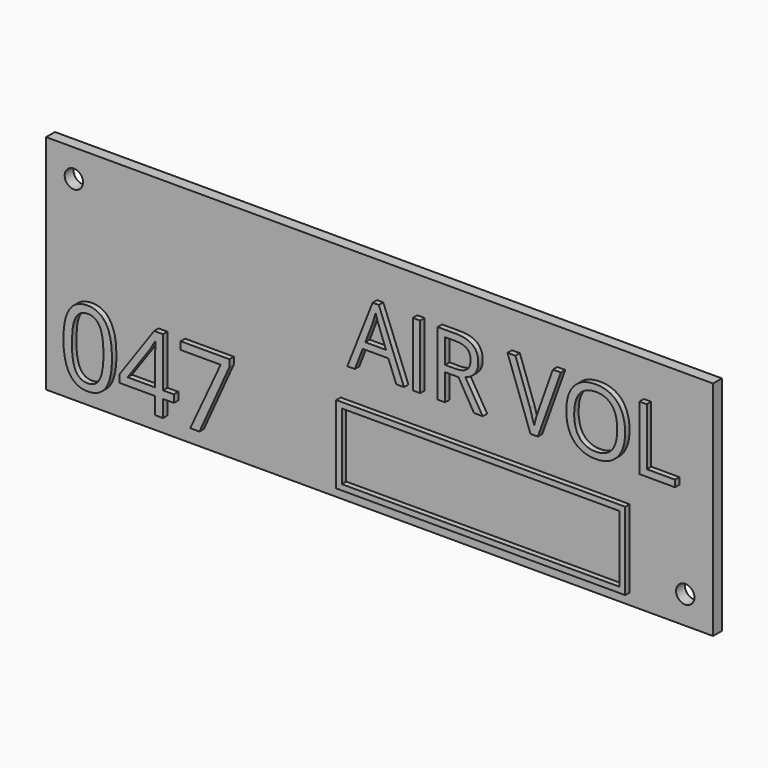
from build123d import *

# Parameters (mm, degrees)
F0_W         = 120
F0_H         = 40
F1_DEPTH     = 2
F3_D         = 3.3
F4_TEXT_SIZE = 16.1100855848
F5_DEPTH     = 1
F6_TEXT_SIZE = 18.5054667028
F7_DEPTH     = 1
F8_W         = 52
F8_H         = 14
F8_W_2       = 49.99999962
F8_H_2       = 11.99999962
F9_DEPTH     = 1


# Not quite as in the source:
# - Text() gives the source's letters only with a copy of the font that has no kerning and outlines rounded to 1/6400 em; it was checked with that copy


with BuildPart() as f1:
    # F0 (on Front) → F1 (new body)
    with BuildSketch(Plane.XZ):
        Rectangle(F0_W, F0_H)
    extrude(amount=F1_DEPTH)

    # F3 (through all)
    with Locations(Plane.XZ.offset(2)):
        with Locations((-55, 15), (55, -15)):
            Hole(F3_D / 2)

    # F4 (on face) → F5 (join)
    with BuildSketch(Plane.XZ.offset(2)):
        with Locations((-5, 2)):
            Text('AIR VOL', F4_TEXT_SIZE, font='Open Sans', text_align=(TextAlign.LEFT, TextAlign.BOTTOM))
    extrude(amount=F5_DEPTH)

    # F6 (on face) → F7 (join)
    with BuildSketch(Plane.XZ.offset(2)):
        with Locations((-57, -17)):
            Text('047', F6_TEXT_SIZE, font='Open Sans', text_align=(TextAlign.LEFT, TextAlign.BOTTOM))
    extrude(amount=F7_DEPTH)

    # F8 (on face) → F9 (join)
    with BuildSketch(Plane.XZ.offset(2)):
        with Locations((19, -11)):
            Rectangle(F8_W, F8_H)
        with Locations((19, -11)):
            Rectangle(F8_W_2, F8_H_2, mode=Mode.SUBTRACT)
    extrude(amount=F9_DEPTH)


solid = f1.part
